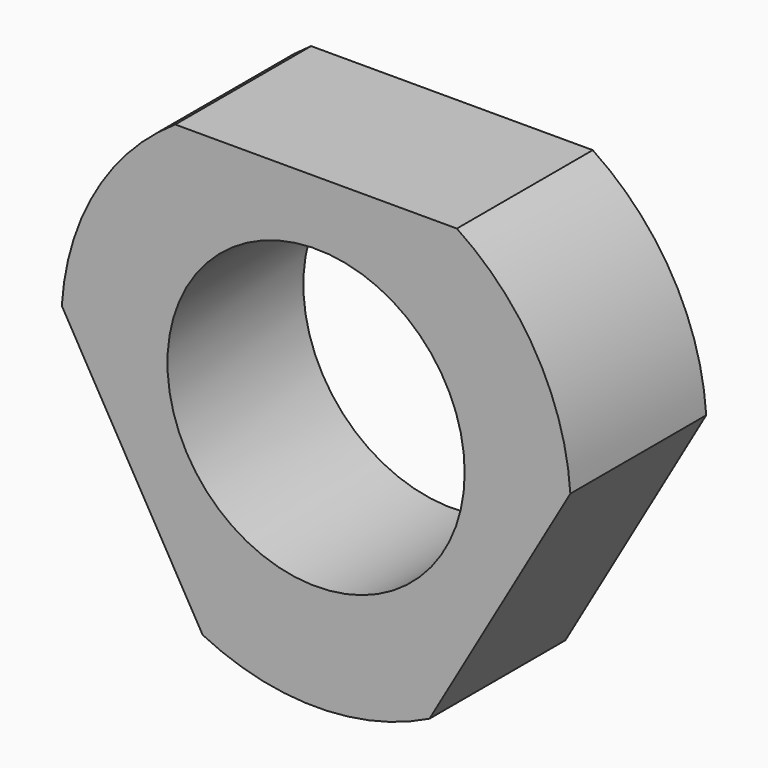
from build123d import *

# Parameters (mm, degrees)
F0_R     = 30
F0_R_2   = 17.5
F1_DEPTH = 20
F2_R     = 100
F3_DEPTH = 20.001


with BuildPart() as f1:
    # F0 (on Front) → F1 (new body)
    with BuildSketch(Plane.XZ):
        Circle(F0_R)
        Circle(F0_R_2, mode=Mode.SUBTRACT)
    extrude(amount=-F1_DEPTH)

    # F2 (on face) → F3 (cut, through all)
    with BuildSketch(Plane.XZ):
        Circle(F2_R)
        with BuildLine():
            ThreePointArc((29.9421970705, 1.8614066163), (29.9855457856, 0.9311519438), (30, 0))
            ThreePointArc((30, 0), (25.5026684247, -15.7991741309), (13.3590731187, -26.8614066163))
            Line((13.3590731187, -26.8614066163), (0, -50))
            Line((0, -50), (-13.3590731187, -26.8614066163))
            ThreePointArc((-13.3590731187, -26.8614066163), (-25.9807621135, -15), (-29.9421970705, 1.8614066163))
            Line((-29.9421970705, 1.8614066163), (-43.3012701892, 25))
            Line((-43.3012701892, 25), (-16.5831239518, 25))
            ThreePointArc((-16.5831239518, 25), (0, 30), (16.5831239518, 25))
            Line((16.5831239518, 25), (43.3012701892, 25))
            Line((43.3012701892, 25), (29.9421970705, 1.8614066163))
        make_face(mode=Mode.SUBTRACT)
        with BuildLine():
            Line((-16.5831239518, 25), (16.5831239518, 25))
            ThreePointArc((16.5831239518, 25), (0, 30), (-16.5831239518, 25))
        make_face()
        with BuildLine():
            ThreePointArc((-29.9421970705, 1.8614066163), (-25.9807621135, -15), (-13.3590731187, -26.8614066163))
            Line((-13.3590731187, -26.8614066163), (-29.9421970705, 1.8614066163))
        make_face()
        with BuildLine():
            ThreePointArc((13.3590731187, -26.8614066163), (25.5026684247, -15.7991741309), (30, 0))
            ThreePointArc((30, 0), (29.9855457856, 0.9311519438), (29.9421970705, 1.8614066163))
            Line((29.9421970705, 1.8614066163), (13.3590731187, -26.8614066163))
        make_face()
    extrude(amount=-F3_DEPTH, mode=Mode.SUBTRACT)


solid = f1.part
